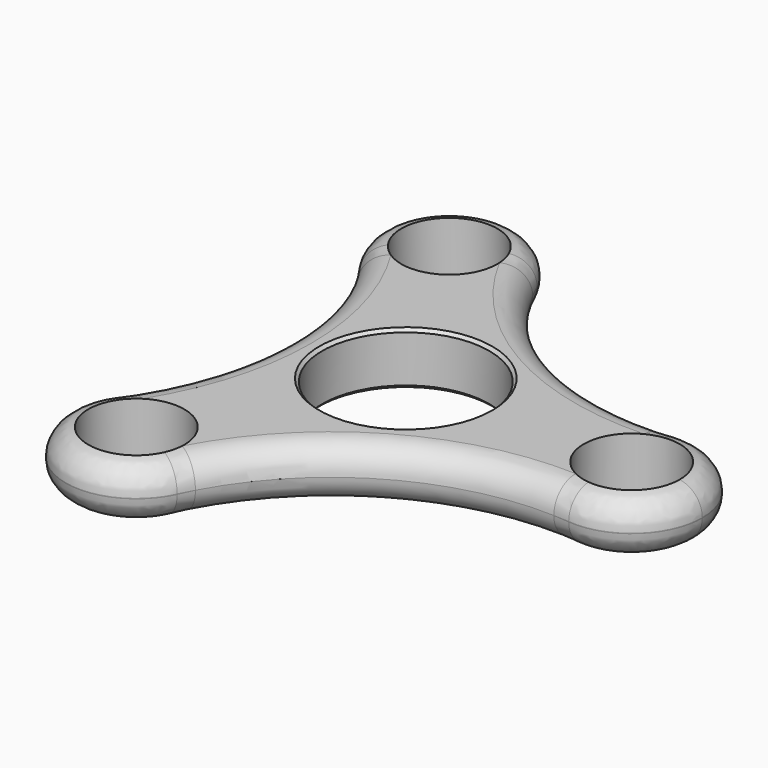
from build123d import *

# Parameters (mm, degrees)
F0_R     = 6.375
F0_R_2   = 11.1
F1_DEPTH = 7
F2_R     = 3.49999
F3_SIZE  = 0.4


# Not quite as in the source:
# - a fillet or chamfer is up to 0.001 mm smaller than in the source, because OpenCascade refuses the exact size
# - a feature names something its author has since deleted; it is built from what else it names


with BuildPart() as f1:
    # F0 (on Top) → F1 (new body)
    with BuildSketch(Plane.XY):
        with BuildLine():
            ThreePointArc((-6.4705763528, -29.8717205104), (8.0319401122, -13.9117283577), (29.1049569931, -9.3321767566))
            ThreePointArc((29.1049569931, -9.3321767566), (39.375, 0), (29.1049569931, 9.3321767566))
            ThreePointArc((29.1049569931, 9.3321767566), (8.0319401122, 13.9117283577), (-6.4705763528, 29.8717205104))
            ThreePointArc((-6.4705763528, 29.8717205104), (-19.6875, 34.099750274), (-22.6343806404, 20.5395437538))
            ThreePointArc((-22.6343806404, 20.5395437538), (-16.0638802244, 0), (-22.6343806404, -20.5395437538))
            ThreePointArc((-22.6343806404, -20.5395437538), (-19.6875, -34.099750274), (-6.4705763528, -29.8717205104))
        make_face()
        with Locations((-15, -25.9807621135)):
            Circle(F0_R, mode=Mode.SUBTRACT)
        Circle(F0_R_2, mode=Mode.SUBTRACT)
        with Locations((-15, 25.9807621135)):
            Circle(F0_R, mode=Mode.SUBTRACT)
        with Locations((30, 0)):
            Circle(F0_R, mode=Mode.SUBTRACT)
    extrude(amount=F1_DEPTH)

    # F2 (radius 3.5 in the source; OpenCascade refuses exactly that, so slightly less here)
    f2_edges = [f1.edges().sort_by_distance(p)[0] for p in [
        (8.03194, -13.911728, 0),
        (8.03194, -13.911728, 7),
    ]]
    fillet(f2_edges, radius=F2_R)

    # F3
    f3_edges = [f1.edges().sort_by_distance(p)[0] for p in [
        (-11.1, 0, 7),
        (-11.1, 0, 0),
    ]]
    chamfer(f3_edges, length=F3_SIZE)


solid = f1.part
